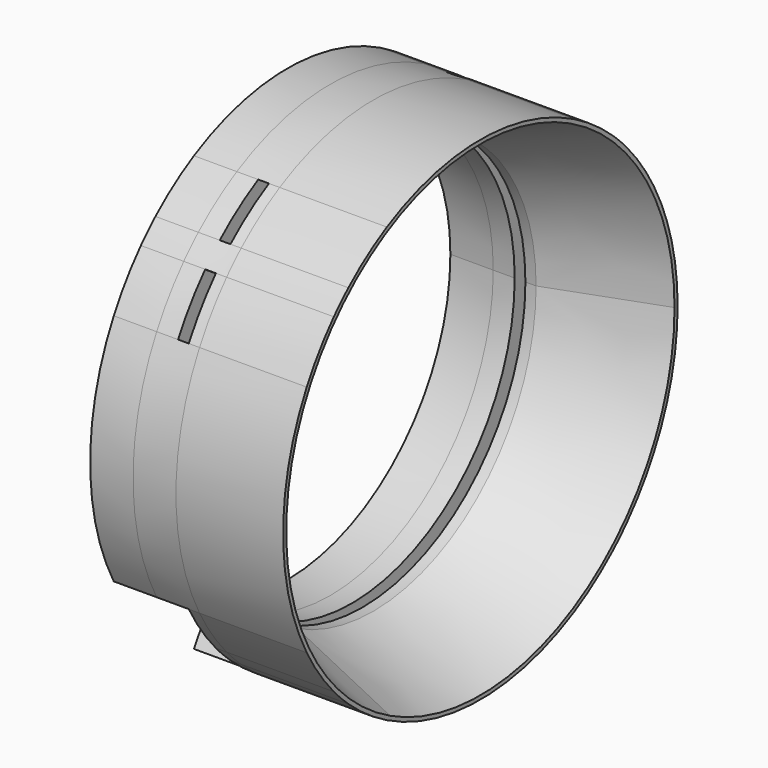
from build123d import *
from build123d import SkipClean  # not in build123d's __all__

# Parameters (mm, degrees)
F1_DEPTH = 4
F2_DEPTH = 3
F3_DEPTH = 2
F4_DEPTH = 4
F5_DEPTH = 10
F6_SIZE2 = 3.639692
F6_SIZE  = 9.99999


# Not quite as in the source:
# - a fillet or chamfer is up to 0.001 mm smaller than in the source, because OpenCascade refuses the exact size


with BuildPart() as f1:
    # F0 (on Right) → F1 (new body)
    with BuildSketch(Plane.YZ):
        with BuildLine():
            ThreePointArc((-10.9058470556, -20.25), (0, -23), (10.9058470556, -20.25))
            Line((10.9058470556, -20.25), (-10.9058470556, -20.25))
        make_face()
        with BuildLine():
            Line((-10.9058470556, -20.25), (10.9058470556, -20.25))
            ThreePointArc((10.9058470556, -20.25), (13.2440741804, -18.8041085698), (15.3930810865, -17.0895598148))
            ThreePointArc((15.3930810865, -17.0895598148), (15.4149278299, -15.4149278299), (17.0895598148, -15.3930810865))
            ThreePointArc((17.0895598148, -15.3930810865), (18.8041085698, -13.2440741804), (20.25, -10.9058470556))
            Line((20.25, -10.9058470556), (20.25, 10.9058470556))
            ThreePointArc((20.25, 10.9058470556), (18.8041085698, 13.2440741804), (17.0895598148, 15.3930810865))
            ThreePointArc((17.0895598148, 15.3930810865), (15.4149278299, 15.4149278299), (15.3930810865, 17.0895598148))
            ThreePointArc((15.3930810865, 17.0895598148), (13.2440741804, 18.8041085698), (10.9058470556, 20.25))
            Line((10.9058470556, 20.25), (-10.9058470556, 20.25))
            ThreePointArc((-10.9058470556, 20.25), (-13.2440741804, 18.8041085698), (-15.3930810865, 17.0895598148))
            ThreePointArc((-15.3930810865, 17.0895598148), (-15.4149278299, 15.4149278299), (-17.0895598148, 15.3930810865))
            ThreePointArc((-17.0895598148, 15.3930810865), (-18.8041085698, 13.2440741804), (-20.25, 10.9058470556))
            Line((-20.25, 10.9058470556), (-20.25, -10.9058470556))
            Line((-20.25, -10.9058470556), (-16.7913530234, -8.8910327658))
            ThreePointArc((-16.7913530234, -8.8910327658), (-4.5806272799, 18.4395730353), (19, 0))
            ThreePointArc((19, 0), (9.8278072985, -16.2608180515), (-8.833074074, -16.8219143501))
            Line((-8.833074074, -16.8219143501), (-10.9058470556, -20.25))
        make_face()
        with BuildLine():
            ThreePointArc((-15.3930810865, -17.0895598148), (-13.2440741804, -18.8041085698), (-10.9058470556, -20.25))
            Line((-10.9058470556, -20.25), (-8.833074074, -16.8219143501))
            ThreePointArc((-8.833074074, -16.8219143501), (-13.4118431505, -13.4581745904), (-16.7913530234, -8.8910327658))
            Line((-16.7913530234, -8.8910327658), (-20.25, -10.9058470556))
            ThreePointArc((-20.25, -10.9058470556), (-18.8041085698, -13.2440741804), (-17.0895598148, -15.3930810865))
            ThreePointArc((-17.0895598148, -15.3930810865), (-15.4149278299, -15.4149278299), (-15.3930810865, -17.0895598148))
        make_face()
        with BuildLine():
            ThreePointArc((17.0895598148, -15.3930810865), (15.4149278299, -15.4149278299), (15.3930810865, -17.0895598148))
            ThreePointArc((15.3930810865, -17.0895598148), (16.2634559673, -16.2634559673), (17.0895598148, -15.3930810865))
        make_face()
        with BuildLine():
            ThreePointArc((-17.0895598148, -15.3930810865), (-16.2634559673, -16.2634559673), (-15.3930810865, -17.0895598148))
            ThreePointArc((-15.3930810865, -17.0895598148), (-15.4149278299, -15.4149278299), (-17.0895598148, -15.3930810865))
        make_face()
        with BuildLine():
            Line((20.25, 10.9058470556), (20.25, -10.9058470556))
            ThreePointArc((20.25, -10.9058470556), (22.3019057482, -5.6236109396), (23, 0))
            ThreePointArc((23, 0), (22.3019057482, 5.6236109396), (20.25, 10.9058470556))
        make_face()
        with BuildLine():
            ThreePointArc((-20.25, 10.9058470556), (-23, 0), (-20.25, -10.9058470556))
            Line((-20.25, -10.9058470556), (-20.25, 10.9058470556))
        make_face()
        with BuildLine():
            ThreePointArc((15.3930810865, 17.0895598148), (15.4149278299, 15.4149278299), (17.0895598148, 15.3930810865))
            ThreePointArc((17.0895598148, 15.3930810865), (16.2634559673, 16.2634559673), (15.3930810865, 17.0895598148))
        make_face()
        with BuildLine():
            ThreePointArc((-15.3930810865, 17.0895598148), (-16.2634559673, 16.2634559673), (-17.0895598148, 15.3930810865))
            ThreePointArc((-17.0895598148, 15.3930810865), (-15.4149278299, 15.4149278299), (-15.3930810865, 17.0895598148))
        make_face()
        with BuildLine():
            Line((-10.9058470556, 20.25), (10.9058470556, 20.25))
            ThreePointArc((10.9058470556, 20.25), (0, 23), (-10.9058470556, 20.25))
        make_face()
    extrude(amount=F1_DEPTH)

    # F0 (on Right) → F2 (cut)
    with BuildSketch(Plane.YZ):
        with BuildLine():
            Line((-10.9058470556, -20.25), (10.9058470556, -20.25))
            ThreePointArc((10.9058470556, -20.25), (13.2440741804, -18.8041085698), (15.3930810865, -17.0895598148))
            ThreePointArc((15.3930810865, -17.0895598148), (15.4149278299, -15.4149278299), (17.0895598148, -15.3930810865))
            ThreePointArc((17.0895598148, -15.3930810865), (18.8041085698, -13.2440741804), (20.25, -10.9058470556))
            Line((20.25, -10.9058470556), (20.25, 10.9058470556))
            ThreePointArc((20.25, 10.9058470556), (18.8041085698, 13.2440741804), (17.0895598148, 15.3930810865))
            ThreePointArc((17.0895598148, 15.3930810865), (15.4149278299, 15.4149278299), (15.3930810865, 17.0895598148))
            ThreePointArc((15.3930810865, 17.0895598148), (13.2440741804, 18.8041085698), (10.9058470556, 20.25))
            Line((10.9058470556, 20.25), (-10.9058470556, 20.25))
            ThreePointArc((-10.9058470556, 20.25), (-13.2440741804, 18.8041085698), (-15.3930810865, 17.0895598148))
            ThreePointArc((-15.3930810865, 17.0895598148), (-15.4149278299, 15.4149278299), (-17.0895598148, 15.3930810865))
            ThreePointArc((-17.0895598148, 15.3930810865), (-18.8041085698, 13.2440741804), (-20.25, 10.9058470556))
            Line((-20.25, 10.9058470556), (-20.25, -10.9058470556))
            Line((-20.25, -10.9058470556), (-16.7913530234, -8.8910327658))
            ThreePointArc((-16.7913530234, -8.8910327658), (-4.5806272799, 18.4395730353), (19, 0))
            ThreePointArc((19, 0), (9.8278072985, -16.2608180515), (-8.833074074, -16.8219143501))
            Line((-8.833074074, -16.8219143501), (-10.9058470556, -20.25))
        make_face()
        with BuildLine():
            ThreePointArc((-15.3930810865, -17.0895598148), (-13.2440741804, -18.8041085698), (-10.9058470556, -20.25))
            Line((-10.9058470556, -20.25), (-8.833074074, -16.8219143501))
            ThreePointArc((-8.833074074, -16.8219143501), (-13.4118431505, -13.4581745904), (-16.7913530234, -8.8910327658))
            Line((-16.7913530234, -8.8910327658), (-20.25, -10.9058470556))
            ThreePointArc((-20.25, -10.9058470556), (-18.8041085698, -13.2440741804), (-17.0895598148, -15.3930810865))
            ThreePointArc((-17.0895598148, -15.3930810865), (-15.4149278299, -15.4149278299), (-15.3930810865, -17.0895598148))
        make_face()
        with BuildLine():
            ThreePointArc((-17.0895598148, -15.3930810865), (-16.2634559673, -16.2634559673), (-15.3930810865, -17.0895598148))
            ThreePointArc((-15.3930810865, -17.0895598148), (-15.4149278299, -15.4149278299), (-17.0895598148, -15.3930810865))
        make_face()
    extrude(amount=F2_DEPTH, mode=Mode.SUBTRACT)


with BuildPart() as f3:
    # F0 (on Right) → F3 (new body)
    with BuildSketch(Plane.YZ):
        with BuildLine():
            Line((-10.9058470556, -20.25), (10.9058470556, -20.25))
            ThreePointArc((10.9058470556, -20.25), (13.2440741804, -18.8041085698), (15.3930810865, -17.0895598148))
            ThreePointArc((15.3930810865, -17.0895598148), (15.4149278299, -15.4149278299), (17.0895598148, -15.3930810865))
            ThreePointArc((17.0895598148, -15.3930810865), (18.8041085698, -13.2440741804), (20.25, -10.9058470556))
            Line((20.25, -10.9058470556), (20.25, 10.9058470556))
            ThreePointArc((20.25, 10.9058470556), (18.8041085698, 13.2440741804), (17.0895598148, 15.3930810865))
            ThreePointArc((17.0895598148, 15.3930810865), (15.4149278299, 15.4149278299), (15.3930810865, 17.0895598148))
            ThreePointArc((15.3930810865, 17.0895598148), (13.2440741804, 18.8041085698), (10.9058470556, 20.25))
            Line((10.9058470556, 20.25), (-10.9058470556, 20.25))
            ThreePointArc((-10.9058470556, 20.25), (-13.2440741804, 18.8041085698), (-15.3930810865, 17.0895598148))
            ThreePointArc((-15.3930810865, 17.0895598148), (-15.4149278299, 15.4149278299), (-17.0895598148, 15.3930810865))
            ThreePointArc((-17.0895598148, 15.3930810865), (-18.8041085698, 13.2440741804), (-20.25, 10.9058470556))
            Line((-20.25, 10.9058470556), (-20.25, -10.9058470556))
            Line((-20.25, -10.9058470556), (-16.7913530234, -8.8910327658))
            ThreePointArc((-16.7913530234, -8.8910327658), (-4.5806272799, 18.4395730353), (19, 0))
            ThreePointArc((19, 0), (9.8278072985, -16.2608180515), (-8.833074074, -16.8219143501))
            Line((-8.833074074, -16.8219143501), (-10.9058470556, -20.25))
        make_face()
    extrude(amount=F3_DEPTH)

    # F0 (on Right) → F4 (join)
    with BuildSketch(Plane.YZ):
        with BuildLine():
            ThreePointArc((-10.9058470556, -20.25), (0, -23), (10.9058470556, -20.25))
            Line((10.9058470556, -20.25), (-10.9058470556, -20.25))
        make_face()
        with BuildLine():
            Line((-10.9058470556, 20.25), (10.9058470556, 20.25))
            ThreePointArc((10.9058470556, 20.25), (0, 23), (-10.9058470556, 20.25))
        make_face()
        with BuildLine():
            Line((20.25, 10.9058470556), (20.25, -10.9058470556))
            ThreePointArc((20.25, -10.9058470556), (22.3019057482, -5.6236109396), (23, 0))
            ThreePointArc((23, 0), (22.3019057482, 5.6236109396), (20.25, 10.9058470556))
        make_face()
        with BuildLine():
            ThreePointArc((-20.25, 10.9058470556), (-23, 0), (-20.25, -10.9058470556))
            Line((-20.25, -10.9058470556), (-20.25, 10.9058470556))
        make_face()
        with BuildLine():
            ThreePointArc((15.3930810865, 17.0895598148), (15.4149278299, 15.4149278299), (17.0895598148, 15.3930810865))
            ThreePointArc((17.0895598148, 15.3930810865), (16.2634559673, 16.2634559673), (15.3930810865, 17.0895598148))
        make_face()
        with BuildLine():
            ThreePointArc((-15.3930810865, 17.0895598148), (-16.2634559673, 16.2634559673), (-17.0895598148, 15.3930810865))
            ThreePointArc((-17.0895598148, 15.3930810865), (-15.4149278299, 15.4149278299), (-15.3930810865, 17.0895598148))
        make_face()
        with BuildLine():
            ThreePointArc((17.0895598148, -15.3930810865), (15.4149278299, -15.4149278299), (15.3930810865, -17.0895598148))
            ThreePointArc((15.3930810865, -17.0895598148), (16.2634559673, -16.2634559673), (17.0895598148, -15.3930810865))
        make_face()
        with BuildLine():
            Line((-10.9058470556, -20.25), (10.9058470556, -20.25))
            ThreePointArc((10.9058470556, -20.25), (13.2440741804, -18.8041085698), (15.3930810865, -17.0895598148))
            ThreePointArc((15.3930810865, -17.0895598148), (15.4149278299, -15.4149278299), (17.0895598148, -15.3930810865))
            ThreePointArc((17.0895598148, -15.3930810865), (18.8041085698, -13.2440741804), (20.25, -10.9058470556))
            Line((20.25, -10.9058470556), (20.25, 10.9058470556))
            ThreePointArc((20.25, 10.9058470556), (18.8041085698, 13.2440741804), (17.0895598148, 15.3930810865))
            ThreePointArc((17.0895598148, 15.3930810865), (15.4149278299, 15.4149278299), (15.3930810865, 17.0895598148))
            ThreePointArc((15.3930810865, 17.0895598148), (13.2440741804, 18.8041085698), (10.9058470556, 20.25))
            Line((10.9058470556, 20.25), (-10.9058470556, 20.25))
            ThreePointArc((-10.9058470556, 20.25), (-13.2440741804, 18.8041085698), (-15.3930810865, 17.0895598148))
            ThreePointArc((-15.3930810865, 17.0895598148), (-15.4149278299, 15.4149278299), (-17.0895598148, 15.3930810865))
            ThreePointArc((-17.0895598148, 15.3930810865), (-18.8041085698, 13.2440741804), (-20.25, 10.9058470556))
            Line((-20.25, 10.9058470556), (-20.25, -10.9058470556))
            Line((-20.25, -10.9058470556), (-16.7913530234, -8.8910327658))
            ThreePointArc((-16.7913530234, -8.8910327658), (-4.5806272799, 18.4395730353), (19, 0))
            ThreePointArc((19, 0), (9.8278072985, -16.2608180515), (-8.833074074, -16.8219143501))
            Line((-8.833074074, -16.8219143501), (-10.9058470556, -20.25))
        make_face()
    with SkipClean():  # cleaning this boolean's faces spoils the solid; the shape is the same uncleaned
        extrude(amount=-F4_DEPTH)


with BuildPart() as f5:
    # F5 (new): a face of the model
    f5_faces = [f1.part.faces().sort_by_distance(p)[0] for p in [
        (4, -10.5973831193, -19.6772435072),
    ]]
    extrude(f5_faces, amount=F5_DEPTH)

    # F6 (size 10 and 3.6397023427 in the source; OpenCascade refuses exactly that, so slightly less here)
    f6_edges = [f5.edges().sort_by_distance(p)[0] for p in [
        (14, 8.833074, 16.821914),
    ]]
    f6_side = f5.faces().sort_by_distance((9, 8.833074, 16.821914))[0]
    chamfer(f6_edges, length=F6_SIZE, length2=F6_SIZE2, reference=f6_side)


solid = Compound([f1.part, f3.part, f5.part])
